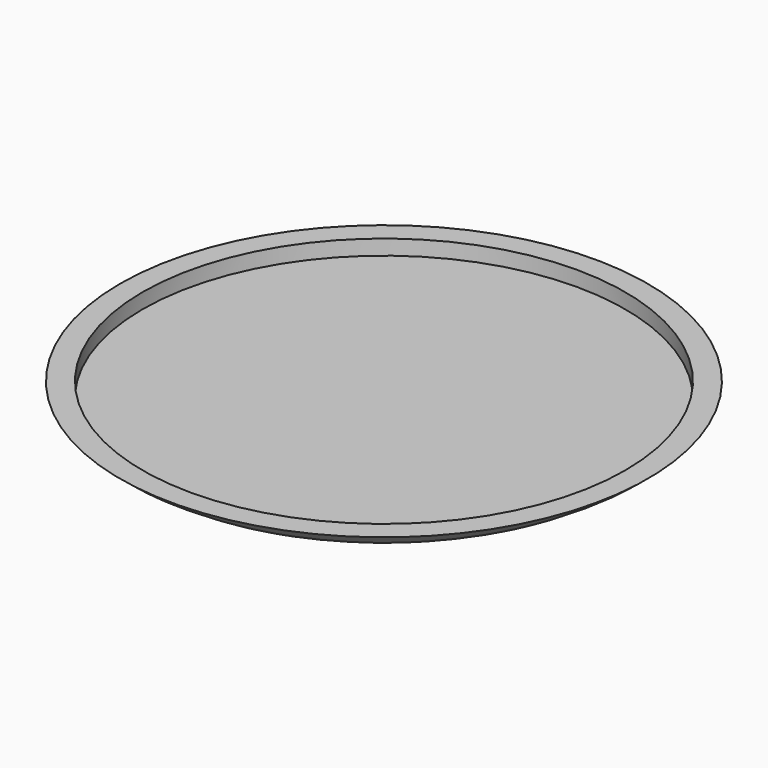
from build123d import *


# Not quite as in the source:
# - a fillet or chamfer that OpenCascade refuses, or shapes differently, is made with other operations: its cross-section is extruded or revolved along the edge and cut away or added


with BuildPart() as f1:
    # F0 (on Front) → F1 (revolve)
    with BuildSketch(Plane.XZ):
        Polygon((-35, 0), (0, 0), (0, 3), (-32, 3), (-32, 5), (-35, 5), align=None)
    revolve(axis=Axis((0, 0, 1.5), (0, 0, -1)))

    # F2: fillet of radius 20 on 1 edges, made by hand

    # F2_s1 → F2_t2 (revolve, cut)
    with BuildSketch(Plane.XZ):
        with BuildLine():
            ThreePointArc((-21.7712434447, 0), (-28.8423112565, 1.2917130661), (-35, 5))
            Line((-35, 5), (-35, 0))
            Line((-35, 0), (-21.7712434447, 0))
        make_face()
    revolve(axis=Axis((0, 0, 0), (0, 0, -1)), mode=Mode.SUBTRACT)


solid = f1.part
